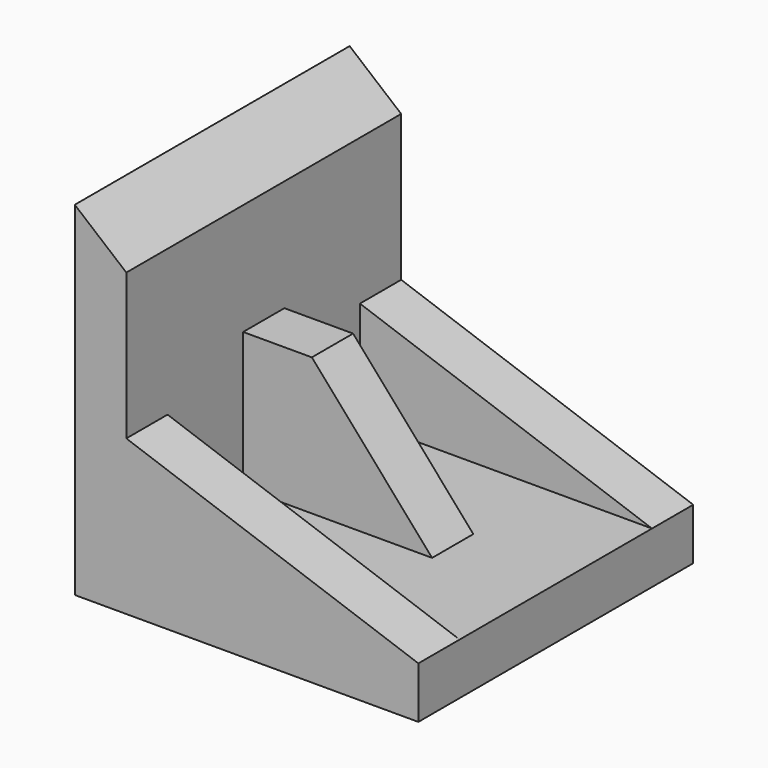
from build123d import *

# Parameters (mm, degrees)
F1_DEPTH = 127
F2_DEPTH = 19.05
F4_DEPTH = 38.1


# Not quite as in the source:
# - a pattern or mirror of a feature is missing from the dataset's text; its kind, count and spacing are read off the source's solid


with BuildPart() as f1:
    # F0 (on Front) → F1 (new body, symmetric)
    with BuildSketch(Plane.XZ):
        Polygon((0, 254), (0, 0), (254, 0), (254, 38.1), (177.8, 38.1), (38.1, 38.1), (38.1, 139.7), (38.1, 222.25), align=None)
    extrude(amount=F1_DEPTH, both=True)

    # F0 (on Front) → F2 (join, symmetric)
    with BuildSketch(Plane.XZ):
        Polygon((38.1, 38.1), (177.8, 38.1), (88.9, 139.7), (38.1, 139.7), align=None)
    extrude(amount=F2_DEPTH, both=True)

    # F3 (on face) → F4 (join)
    with BuildSketch(Plane.XZ.offset(127)):
        Polygon((254, 38.1), (38.1, 114.3), (38.1, 38.1), align=None)
    f4 = extrude(amount=-F4_DEPTH)

    # F4_copies: F4 across plane
    add(f4.mirror(Plane.ZX))


solid = f1.part
